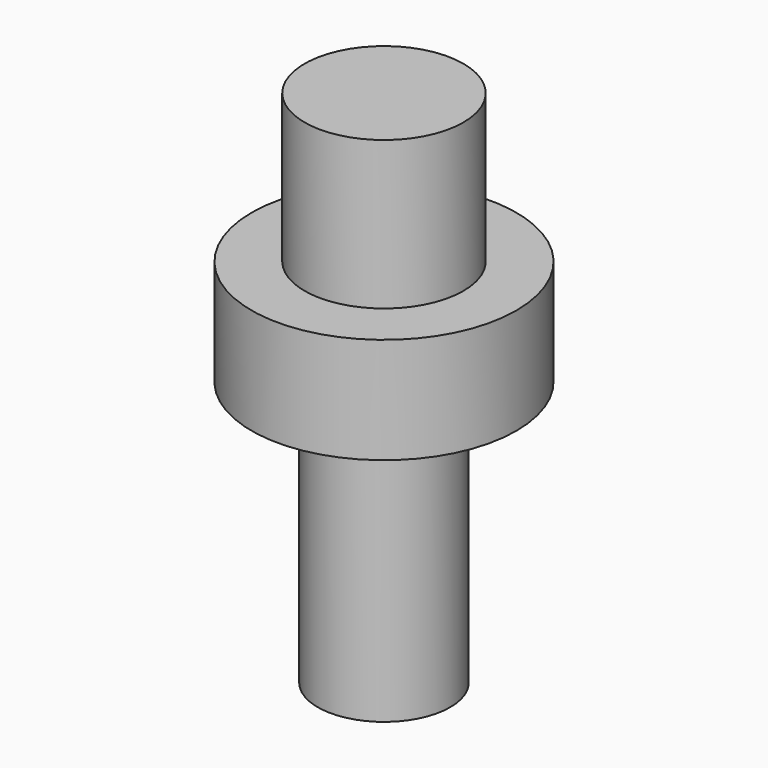
from build123d import *

# Parameters (mm, degrees)
F0_R     = 1.5
F1_DEPTH = 2.8
F2_R     = 2.5
F2_R_2   = 1.5
F3_DEPTH = 2
F4_R     = 1.25
F5_DEPTH = 5


with BuildPart() as f1:
    # F0 (on Top) → F1 (new body)
    with BuildSketch(Plane.XY):
        Circle(F0_R)
    extrude(amount=F1_DEPTH)

    # F2 (on face) → F3 (join)
    with BuildSketch(Plane(origin=(0, 0, 0), x_dir=(1, 0, 0), z_dir=(0, 0, -1))):
        Circle(F2_R)
        Circle(F2_R_2, mode=Mode.SUBTRACT)
        Circle(F2_R_2)
    extrude(amount=F3_DEPTH)

    # F4 (on face) → F5 (join)
    with BuildSketch(Plane(origin=(0, 0, -2), x_dir=(1, 0, 0), z_dir=(0, 0, -1))):
        Circle(F4_R)
    extrude(amount=F5_DEPTH)


solid = f1.part
